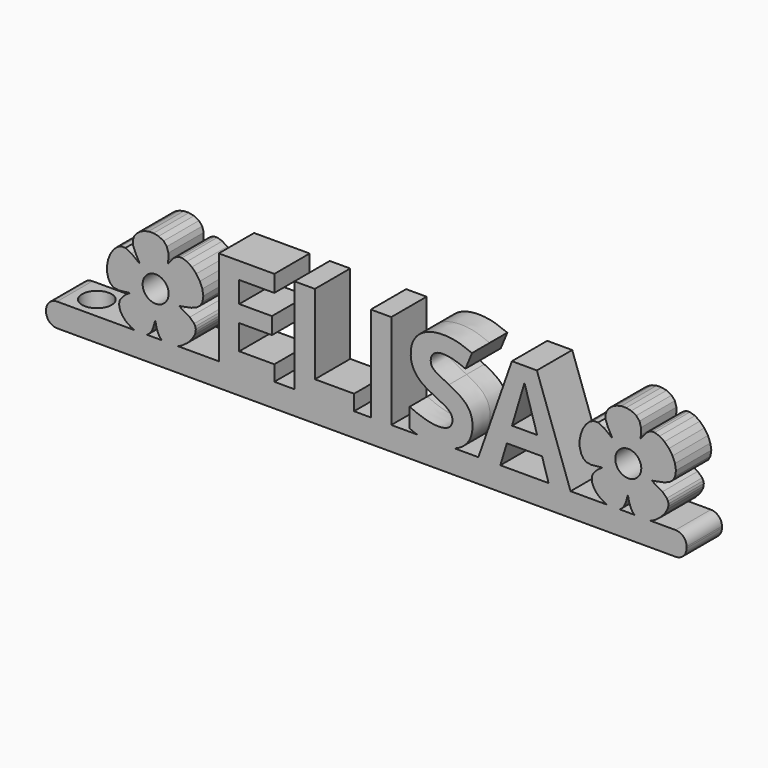
from build123d import *

# Parameters (mm, degrees)
F0_R         = 1.7660260944
F0_TEXT_SIZE = 18.3551006001
F1_DEPTH     = 3
F2_W         = 79.5
F2_H         = 6
F3_DEPTH     = 0.2
F4_DEPTH     = 3
F5_W         = 6
F5_H         = 3.2
F6_DEPTH     = 7.5
F7_R         = 1.5
F8_R         = 2
F9_DEPTH     = 4
F10_R        = 1.5


# Not quite as in the source:
# - Text() gives the source's letters only with a copy of the font that has no kerning and outlines rounded to 1/6400 em; it was checked with that copy


with BuildPart() as f1:
    # F0 (on Front) → F1 (new body, symmetric)
    with BuildSketch(Plane.XZ):
        Polygon((-9.8962181259, -0.0299609487), (-9.3093152472, 0.0995427735), (-8.5310452338, 0.4643787281), (-7.7886221935, 1.0156229815), (-7.1753136859, 1.6703047867), (-6.7844076966, 2.345448762), (-6.6844409889, 2.697736103), (-6.6652413988, 3.0240118702), (-6.7312263226, 3.3305926174), (-6.8868132072, 3.6238062576), (-7.4844896445, 4.1953846804), (-8.4936258745, 4.789299945), (-8.9274018823, 5.0567831788), (-8.4181052429, 5.1580766137), (-7.3131137554, 5.3695361907), (-6.5480905692, 5.6521941874), (-6.0523445823, 6.043851435), (-5.7552051187, 6.5823041299), (-5.6420905942, 7.3346827833), (-5.7751165223, 8.1369112107), (-6.1089634595, 8.9328581362), (-6.5983028952, 9.6663968681), (-7.1978267956, 10.281407439), (-7.8622157172, 10.7217585729), (-8.546147975, 10.9313258196), (-8.8812811082, 10.9320270148), (-9.2043064176, 10.8539824368), (-9.6469000392, 10.5612860557), (-10.1400767255, 9.9810366231), (-10.4508130024, 9.5801644376), (-10.4068223535, 10.0271686751), (-10.3916193646, 10.9311557532), (-10.598433195, 11.6324207168), (-11.0363252865, 12.1480644274), (-11.7143548393, 12.4951945719), (-12.3982545289, 12.6383143795), (-13.0712303381, 12.6247535348), (-13.7032208938, 12.4733707309), (-14.2641853, 12.2030313855), (-14.7240621838, 11.8325941916), (-15.0528129411, 11.3809291004), (-15.2203761991, 10.8668948051), (-15.1967042361, 10.3093544817), (-14.8286469794, 9.4077545862), (-14.3529716358, 8.5454741101), (-14.2906102139, 8.4004774316), (-14.4811582303, 8.5293860258), (-15.3946726039, 9.2300894295), (-16.21802192, 9.6332437342), (-16.8030362894, 9.634121823), (-17.3568401554, 9.3699870508), (-17.8525159958, 8.8932532172), (-18.2631576982, 8.2563454299), (-18.5618432066, 7.5116797807), (-18.7216618753, 6.7116836696), (-18.7156984739, 5.9087754295), (-18.5170445979, 5.1553756349), (-18.2008868091, 4.6439944488), (-17.7512302174, 4.3560670179), (-17.1086136552, 4.2712956407), (-16.2135760559, 4.3694053341), (-15.7044514474, 4.4302814773), (-15.6696932647, 4.4000047008), (-15.7790195709, 4.3290260096), (-16.1651405309, 4.0708069691), (-16.5523139664, 3.7127982689), (-16.8671052824, 3.3322639471), (-17.0360798838, 3.0064680418), (-17.0831036318, 2.6043628391), (-17.0239245605, 2.1921008316), (-16.867618816, 1.7819255621), (-16.6232807801, 1.3860941234), (-16.3000002503, 1.0168545414), (-15.9068693162, 0.6864593752), (-15.4529754831, 0.4071521172), (-14.9474063577, 0.1911989779), (-14.4397479673, 0.0570083052), (-13.9840845603, 0.0188926715), (-13.5797273957, 0.0772799851), (-13.2259605822, 0.2326232662), (-12.9220907946, 0.485341356), (-12.6674066752, 0.8358849825), (-12.4612081239, 1.2846821047), (-12.3027905578, 1.8321743328), (-12.1879723822, 2.2557758958), (-12.1309056827, 2.0998483864), (-12.0112204133, 1.5291342486), (-11.8237778137, 0.9902805659), (-11.5954117235, 0.5466869075), (-11.3529559319, 0.2617414835), (-10.9521058183, 0.053843468), (-10.4551700276, -0.0442881949), align=None)
        with Locations((-12.1185852993, 6.0541479067)):
            Circle(F0_R, mode=Mode.SUBTRACT)
        Polygon((54.0599232745, 9.9810366231), (53.7491869976, 9.5801644376), (53.7931776465, 10.0271686751), (53.8083806354, 10.9311557532), (53.601566805, 11.6324207168), (53.1636747135, 12.1480644274), (52.4856451607, 12.4951945719), (51.8017454711, 12.6383143795), (51.1287696619, 12.6247535348), (50.4967791062, 12.4733707309), (49.9358147, 12.2030313855), (49.4759378162, 11.8325941916), (49.1471870589, 11.3809291004), (48.9796238009, 10.8668948051), (49.0032957639, 10.3093544817), (49.3713530206, 9.4077545862), (49.8470283642, 8.5454741101), (49.9093897861, 8.4004774316), (49.7188417697, 8.5293860258), (48.8053273961, 9.2300894295), (47.98197808, 9.6332437342), (47.3969637106, 9.634121823), (46.8431598446, 9.3699870508), (46.3474840042, 8.8932532172), (45.9368423018, 8.2563454299), (45.6381567934, 7.5116797807), (45.4783381247, 6.7116836696), (45.4843015261, 5.9087754295), (45.6829554021, 5.1553756349), (45.9991131909, 4.6439944488), (46.4487697826, 4.3560670179), (47.0913863448, 4.2712956407), (47.9864239441, 4.3694053341), (48.4955485526, 4.4302814773), (48.5303067353, 4.4000047008), (48.4209804291, 4.3290260096), (48.0348594691, 4.0708069691), (47.6476860336, 3.7127982689), (47.3328947176, 3.3322639471), (47.1639201162, 3.0064680418), (47.1168963682, 2.6043628391), (47.1760754395, 2.1921008316), (47.332381184, 1.7819255621), (47.5767192199, 1.3860941234), (47.8999997497, 1.0168545414), (48.2931306838, 0.6864593752), (48.7470245169, 0.4071521172), (49.2525936423, 0.1911989779), (49.7602520327, 0.0570083052), (50.2159154397, 0.0188926715), (50.6202726043, 0.0772799851), (50.9740394178, 0.2326232662), (51.2779092054, 0.485341356), (51.5325933248, 0.8358849825), (51.7387918761, 1.2846821047), (51.8972094422, 1.8321743328), (52.0120276178, 2.2557758958), (52.0690943173, 2.0998483864), (52.1887795867, 1.5291342486), (52.3762221863, 0.9902805659), (52.6045882765, 0.5466869075), (52.8470440681, 0.2617414835), (53.2478941817, 0.053843468), (53.7448299724, -0.0442881949), (54.3037818741, -0.0299609487), (54.8906847528, 0.0995427735), (55.6689547662, 0.4643787281), (56.4113778065, 1.0156229815), (57.0246863141, 1.6703047867), (57.4155923034, 2.345448762), (57.5155590111, 2.697736103), (57.5347586012, 3.0240118702), (57.4687736774, 3.3305926174), (57.3131867928, 3.6238062576), (56.7155103555, 4.1953846804), (55.7063741255, 4.789299945), (55.2725981177, 5.0567831788), (55.7818947571, 5.1580766137), (56.8868862446, 5.3695361907), (57.6519094308, 5.6521941874), (58.1476554177, 6.043851435), (58.4447948813, 6.5823041299), (58.5579094058, 7.3346827833), (58.4248834777, 8.1369112107), (58.0910365405, 8.9328581362), (57.6016971048, 9.6663968681), (57.0021732044, 10.281407439), (56.3377842828, 10.7217585729), (55.653852025, 10.9313258196), (55.3187188918, 10.9320270148), (54.9956935824, 10.8539824368), (54.5530999608, 10.5612860557), align=None)
        with Locations((52.0814147007, 6.0541479067)):
            Circle(F0_R, mode=Mode.SUBTRACT)
        with Locations((-5.1916254854, 0)):
            Text('ELISA', F0_TEXT_SIZE, font='Open Sans', font_style=FontStyle.BOLD, text_align=(TextAlign.LEFT, TextAlign.BOTTOM))
    extrude(amount=F1_DEPTH, both=True)



with BuildPart() as f3:
    # F2 (on Top) → F3 (new body)
    with BuildSketch(Plane.XY):
        with Locations((20.25, 0)):
            Rectangle(F2_W, F2_H)
    extrude(amount=F3_DEPTH)


with BuildPart() as f4:
    # F4 (new): a face of the model
    f4_faces = [f3.part.faces().sort_by_distance(p)[0] for p in [
        (20.25, 0, 0),
    ]]
    extrude(f4_faces, amount=F4_DEPTH)


with BuildPart() as f1_1:
    add(f1.part)

    add(f3.part)  # F6 merges F3

    add(f4.part)  # F6 merges F4
    # F5 (on face) → F6 (join)
    with BuildSketch(Plane(origin=(-19.5, 0, 0), x_dir=(0, -1, 0), z_dir=(-1, 0, 0))):
        with Locations((0, -1.4)):
            Rectangle(F5_W, F5_H)
    extrude(amount=F6_DEPTH)

    # F7
    f7_edges = [f1_1.edges().sort_by_distance(p)[0] for p in [
        (-27, 0, -3),
        (-27, 0, 0.2),
        (60, 0, -3),
    ]]
    fillet(f7_edges, radius=F7_R)

    # F8 (on face) → F9 (cut)
    with BuildSketch(Plane.XY.offset(0.2)):
        with Locations((-22.5, 0)):
            Circle(F8_R)
    extrude(amount=-F9_DEPTH, mode=Mode.SUBTRACT)

    # F10
    f10_edges = [f1_1.edges().sort_by_distance(p)[0] for p in [
        (60, 0, 0.2),
    ]]
    fillet(f10_edges, radius=F10_R)


solid = f1_1.part
